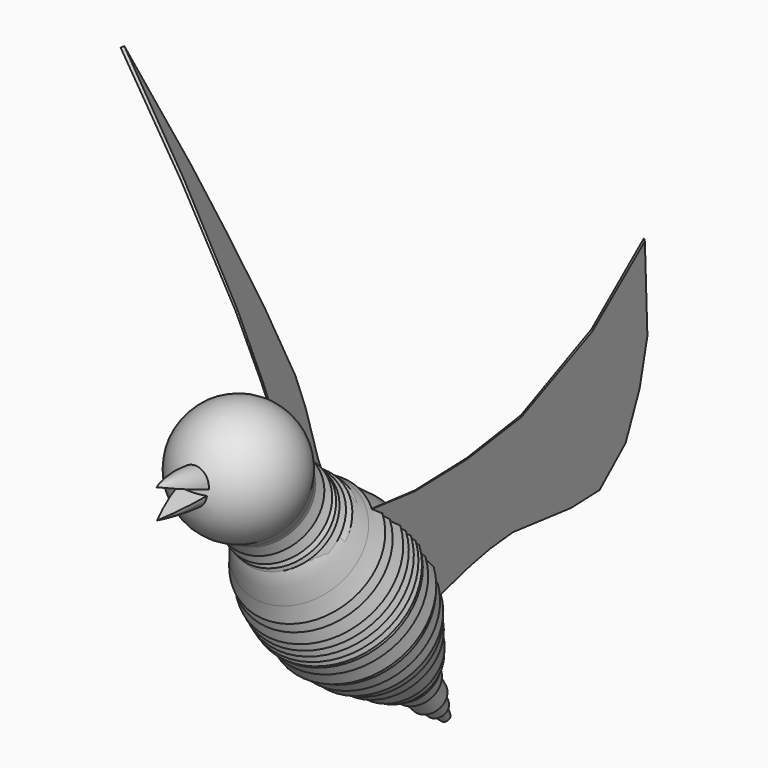
from build123d import *

# Parameters (mm, degrees)
F5_ANGLE_BACK = 90
F5_ANGLE      = 180
F6_ANGLE_BACK = 90
F6_ANGLE      = 180
F8_ANGLE_BACK = 45
F8_ANGLE      = 90
F9_ANGLE_BACK = 44.5
F9_ANGLE      = 89
F10_R         = 0.0254


# Not quite as in the source:
# - a feature names something its author has since deleted; it is built from what else it names


with BuildPart() as f1:
    # F0 (on Right) → F1 (revolve)
    with BuildSketch(Plane.YZ):
        with BuildLine():
            Line((5.1531572826, 8.0174868926), (2.8674317813, 9.2117871624))
            add(Edge.make_bspline(
                [(2.8674317813, 9.2117871624), (-4.9678501465, 14.2756802549), (-9.342409584, 10.8070805006)],
                knots=[2.1366882472, 2.1366882472, 2.1366882472, 3.1415926536, 3.1415926536, 3.1415926536], degree=2, weights=[1, 0.8764042756, 1]))
            Line((-9.342409584, 10.8070805006), (14.3290487186, -19.0470994719))
            Line((14.3290487186, -19.0470994719), (22.8154044598, -29.7499969602))
            Line((22.8154044598, -29.7499969602), (23.2347566634, -29.2056221515))
            Line((23.2347566634, -29.2056221515), (21.9963230193, -26.7373099923))
            Line((21.9963230193, -26.7373099923), (22.448099622, -26.938453486))
            Line((22.448099622, -26.938453486), (21.061127201, -24.3154261261))
            Line((21.061127201, -24.3154261261), (21.5184092522, -24.3154261261))
            Line((21.5184092522, -24.3154261261), (19.4974702676, -21.1042817682))
            Line((19.4974702676, -21.1042817682), (19.9684873223, -21.1042817682))
            Line((19.9684873223, -21.1042817682), (18.5471558688, -18.4162749748))
            Line((18.5471558688, -18.4162749748), (19.1398393363, -18.5852646828))
            Line((19.1398393363, -18.5852646828), (18.3506513549, -15.9694467017))
            Line((18.3506513549, -15.9694467017), (18.952826038, -16.4905972779))
            Line((18.952826038, -16.4905972779), (17.8171513464, -14.1813897826))
            Line((17.8171513464, -14.1813897826), (18.5539294034, -14.8190325126))
            Line((18.5539294034, -14.8190325126), (17.1663262184, -12.0439193743))
            Line((17.1663262184, -12.0439193743), (16.6883822531, -10.4597411454))
            Line((16.6883822531, -10.4597411454), (17.4129810184, -11.1780827865))
            Line((17.4129810184, -11.1780827865), (16.1197113453, -8.5748422102))
            Line((16.1197113453, -8.5748422102), (16.6883822531, -8.9721912518))
            Line((16.6883822531, -8.9721912518), (15.2464192361, -5.9661139308))
            Line((15.2464192361, -5.9661139308), (16.217531725, -7.1217714228))
            Line((16.217531725, -7.1217714228), (15.0355827949, -5.4502797664))
            add(Edge.make_bspline(
                [(15.0355827949, -5.4502797664), (14.7526554069, -4.7776191285), (14.4272786492, -4.1026814411)],
                knots=[1.088548679, 1.088548679, 1.088548679, 1.1717906865, 1.1717906865, 1.1717906865], degree=2, weights=[1, 0.9991339711, 1]))
            Line((14.4272786492, -4.1026814411), (15.2464192361, -4.9511841498))
            Line((15.2464192361, -4.9511841498), (13.640389273, -2.5800023672))
            Line((13.640389273, -2.5800023672), (14.1929908888, -3.0310826419))
            Line((14.1929908888, -3.0310826419), (12.8381073443, -1.1488646294))
            Line((12.8381073443, -1.1488646294), (13.9127867991, -1.8152391107))
            Line((13.9127867991, -1.8152391107), (11.8173022894, 0.3553581118))
            Line((11.8173022894, 0.3553581118), (12.4525045976, 0))
            Line((12.4525045976, 0), (10.9368613231, 1.5699715586))
            Line((10.9368613231, 1.5699715586), (11.381983757, 1.5699715586))
            Line((11.381983757, 1.5699715586), (10.4544342266, 2.192379395))
            Line((10.4544342266, 2.192379395), (11.1069483683, 2.2148620337))
            Line((11.1069483683, 2.2148620337), (9.7826179202, 3.014264277))
            Line((9.7826179202, 3.014264277), (10.4641011169, 3.014264277))
            Line((10.4641011169, 3.014264277), (9.0277861587, 3.8812634473))
            Line((9.0277861587, 3.8812634473), (9.6773298049, 3.8812634473))
            Line((9.6773298049, 3.8812634473), (8.192799144, 4.7773669405))
            Line((8.192799144, 4.7773669405), (8.832487586, 4.7773669405))
            Line((8.832487586, 4.7773669405), (7.2049392145, 5.759799853))
            Line((7.2049392145, 5.759799853), (7.9036029056, 5.759799853))
            Line((7.9036029056, 5.759799853), (5.8808368251, 6.9559253752))
            Line((5.8808368251, 6.9559253752), (6.3240762456, 6.9559253752))
            Line((6.3240762456, 6.9559253752), (4.5654393993, 8.0174868926))
            Line((4.5654393993, 8.0174868926), (5.1531572826, 8.0174868926))
        make_face()
    revolve(axis=Axis((0, 2.4933195673, -4.1200094856), (0, 0.6212981182, -0.7835742775)))

    # F7 (on Right) → F8 (revolve)
    with BuildSketch(Plane.YZ, mode=Mode.PRIVATE) as f8_sk:
        Polygon((8.247789837, 12.1281187165), (3.5712819081, 8.603585884), (8.7069310248, 4.7576981597), (10.6027973816, 2.3807911202), (12.196149677, 0), (13.7787386775, -1.607461716), (16.109501943, -7.0950593799), (18.4070188552, -1.607461716), (19.9790019542, 1.4903947012), (21.9175089151, 4.4704480097), (27.7451782377, 8.8625739672), (30.3188115358, 12.1281187165), (31.2074742752, 20.7586199882), (30.3188115358, 30.6882560253), (28.7555512041, 40.3894744813), (23.9706914872, 57.8002855182), (21.9175089151, 41.2116966415), (17.4588318914, 25.6063379347), (12.9653252661, 17.940942198), align=None)
    revolve(f8_sk.sketch.rotate(Axis((0, 0, 0), (0, 0.6018728944, -0.7985918976)), -F8_ANGLE_BACK), axis=Axis((0, 0, 0), (0, 0.6018728944, -0.7985918976)), revolution_arc=F8_ANGLE)

    # F7 (on Right) → F9 (revolve, cut)
    with BuildSketch(Plane.YZ, mode=Mode.PRIVATE) as f9_sk:
        Polygon((8.247789837, 12.1281187165), (3.5712819081, 8.603585884), (8.7069310248, 4.7576981597), (10.6027973816, 2.3807911202), (12.196149677, 0), (13.7787386775, -1.607461716), (16.109501943, -7.0950593799), (18.4070188552, -1.607461716), (19.9790019542, 1.4903947012), (21.9175089151, 4.4704480097), (27.7451782377, 8.8625739672), (30.3188115358, 12.1281187165), (31.2074742752, 20.7586199882), (30.3188115358, 30.6882560253), (28.7555512041, 40.3894744813), (23.9706914872, 57.8002855182), (21.9175089151, 41.2116966415), (17.4588318914, 25.6063379347), (12.9653252661, 17.940942198), align=None)
    revolve(f9_sk.sketch.rotate(Axis((0, 0, 0), (0, 0.6018728944, -0.7985918976)), -F9_ANGLE_BACK), axis=Axis((0, 0, 0), (0, 0.6018728944, -0.7985918976)), revolution_arc=F9_ANGLE, mode=Mode.SUBTRACT)

    # F10
    f10_edges = [f1.edges().sort_by_distance(p)[0] for p in [
        (0, 9.249145, -22.196821),
        (0, 10.415607, -22.261164),
        (0, 12.753203, -23.010315),
        (0, 22.189762, -30.034201),
        (0, 15.153775, -24.548409),
        (0, 17.923881, -26.802957),
        (0, 20.068784, -28.265661),
        (0, 15.046394, -25.007022),
        (0, 12.782625, -23.625917),
        (0, 10.785752, -22.966292),
        (0, 17.819631, -27.248197),
        (0, 20.161636, -28.751396),
    ]]
    fillet(f10_edges, radius=F10_R)


with BuildPart() as f3:
    # F2 (on Right) → F3 (revolve)
    with BuildSketch(Plane.YZ):
        with BuildLine():
            ThreePointArc((-9.2336770975, 10.9022777354), (-7.053343705, 13.8292899626), (-6.280333138, 17.3963207928))
            ThreePointArc((-6.280333138, 17.3963207928), (-6.292919367, 17.8618736598), (-6.3306412842, 18.3260664453))
            ThreePointArc((-6.3306412842, 18.3260664453), (-11.7587755997, 25.4210579334), (-20.5599415445, 23.8903638502))
            Line((-20.5599415445, 23.8903638502), (-9.2336770975, 10.9022777354))
        make_face()
        with BuildLine():
            ThreePointArc((-6.3306412842, 18.3260664453), (-6.292919367, 17.8618736598), (-6.280333138, 17.3963207928))
            ThreePointArc((-6.280333138, 17.3963207928), (-7.053343705, 13.8292899626), (-9.2336770975, 10.9022777354))
            Line((-9.2336770975, 10.9022777354), (0.9147537057, 10.1317800581))
            Line((0.9147537057, 10.1317800581), (1.6607183374, 10.0937889587))
            Line((1.6607183374, 10.0937889587), (0.5429651474, 10.4806693271))
            Line((0.5429651474, 10.4806693271), (0.8503185079, 10.4806693271))
            Line((0.8503185079, 10.4806693271), (0, 10.8940749007))
            Line((0, 10.8940749007), (-0.260625072, 11.0925109475))
            Line((-0.260625072, 11.0925109475), (0.5429651474, 11.0925109475))
            Line((0.5429651474, 11.0925109475), (-0.9304223572, 11.6024846211))
            Line((-0.9304223572, 11.6024846211), (-0.3701218811, 11.6024846211))
            Line((-0.3701218811, 11.6024846211), (-1.920239518, 12.35611666))
            Line((-1.920239518, 12.35611666), (-1.3606260305, 12.35611666))
            Line((-1.3606260305, 12.35611666), (-2.9088430564, 13.1088246649))
            Line((-2.9088430564, 13.1088246649), (-1.9917223151, 13.1088246649))
            Line((-1.9917223151, 13.1088246649), (-3.6732687149, 13.6908469722))
            Line((-3.6732687149, 13.6908469722), (-2.7125195326, 13.9371918864))
            Line((-2.7125195326, 13.9371918864), (-4.6065561473, 15.0365177542))
            Line((-4.6065561473, 15.0365177542), (-4.0277345106, 15.2125917375))
            Line((-4.0277345106, 15.2125917375), (-5.3881970234, 16.3656920195))
            Line((-5.3881970234, 16.3656920195), (-5.8001331054, 17.1109735966))
            Line((-5.8001331054, 17.1109735966), (-6.3306412842, 18.3260664453))
        make_face()
    revolve(axis=Axis((0, -14.896809321, 17.3963207928), (0, -0.6572445746, 0.7536773641)))

    # F4 (on Right) → F5 (revolve)
    with BuildSketch(Plane.YZ, mode=Mode.PRIVATE) as f5_sk:
        with BuildLine():
            ThreePointArc((-21.8501526059, 20.8347838469), (-25.7943092004, 21.3684429366), (-29.7659616917, 21.1093295366))
            Line((-29.7659616917, 21.1093295366), (-22.5507529889, 18.6328977638))
            Line((-22.5507529889, 18.6328977638), (-21.8501526059, 20.8347838469))
        make_face()
    revolve(f5_sk.sketch.rotate(Axis((0, -26.1583573403, 19.8711136502), (0, 0.9458394824, -0.3246346769)), -F5_ANGLE_BACK), axis=Axis((0, -26.1583573403, 19.8711136502), (0, 0.9458394824, -0.3246346769)), revolution_arc=F5_ANGLE)

    # F4 (on Right) → F6 (revolve)
    with BuildSketch(Plane.YZ, mode=Mode.PRIVATE) as f6_sk:
        with BuildLine():
            Line((-21.9554570535, 18.2515831942), (-29.7091193497, 16.8284662068))
            ThreePointArc((-29.7091193497, 16.8284662068), (-25.970293473, 16.1933045482), (-22.1855584532, 15.9524101764))
            Line((-22.1855584532, 15.9524101764), (-21.9554570535, 18.2515831942))
        make_face()
    revolve(f6_sk.sketch.rotate(Axis((0, -25.8322882016, 17.5400247005), (0, 0.9835702622, 0.1805257303)), -F6_ANGLE_BACK), axis=Axis((0, -25.8322882016, 17.5400247005), (0, 0.9835702622, 0.1805257303)), revolution_arc=F6_ANGLE)


solid = Compound([f1.part, f3.part])
